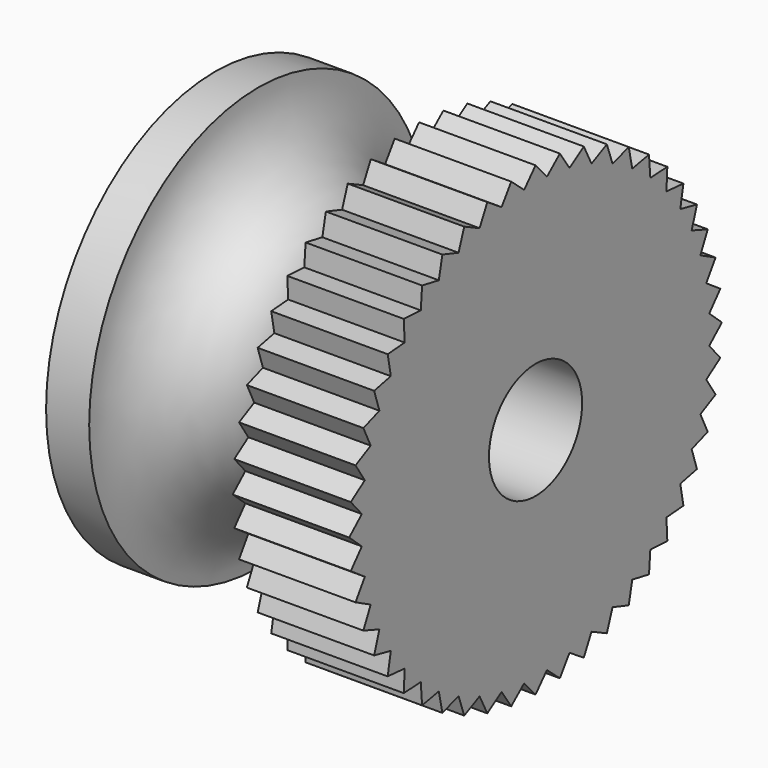
from build123d import *

# Parameters (mm, degrees)
F4_DEPTH        = 3.175
F4_COPIES_COUNT = 48


# Not quite as in the source:
# - a pattern or mirror of a feature is missing from the dataset's text; its kind, count and spacing are read off the source's solid


with BuildPart() as f2:
    # F1 (on offset) → F2 (revolve)
    with BuildSketch(Plane.XZ.offset(60.325)):
        with BuildLine():
            Line((19.05, 5.762625), (19.05, 1.5875))
            Line((19.05, 1.5875), (27.78125, 1.5875))
            Line((27.78125, 1.5875), (27.78125, 6.35))
            Line((27.78125, 6.35), (24.60625, 6.35))
            Line((24.60625, 6.35), (24.60625, 5.762625))
            ThreePointArc((24.60625, 5.762625), (22.4155, 3.571875), (20.22475, 5.762625))
            Line((20.22475, 5.762625), (19.05, 5.762625))
        make_face()
    revolve(axis=Axis((0, -60.325, 0), (1, 0, 0)))

    # F3 (on face) → F4 (cut, through all)
    with BuildSketch(Plane.YZ.offset(27.78125)):
        with BuildLine():
            ThreePointArc((-59.4961586794, 6.2956748697), (-59.9096901294, 6.3364041626), (-60.325, 6.35))
            Line((-60.325, 6.35), (-59.9371006784, 5.9182))
            Line((-59.9371006784, 5.9182), (-59.4961586794, 6.2956748697))
        make_face()
    f4 = extrude(amount=-F4_DEPTH, mode=Mode.SUBTRACT)

    # F4_copies: F4 ×48 about axis
    f4_copies_axis = Axis((0, -60.325, 0), (1, 0, 0))
    for i in range(1, F4_COPIES_COUNT):
        add(f4.rotate(f4_copies_axis, i * 360 / F4_COPIES_COUNT), mode=Mode.SUBTRACT)


solid = f2.part
